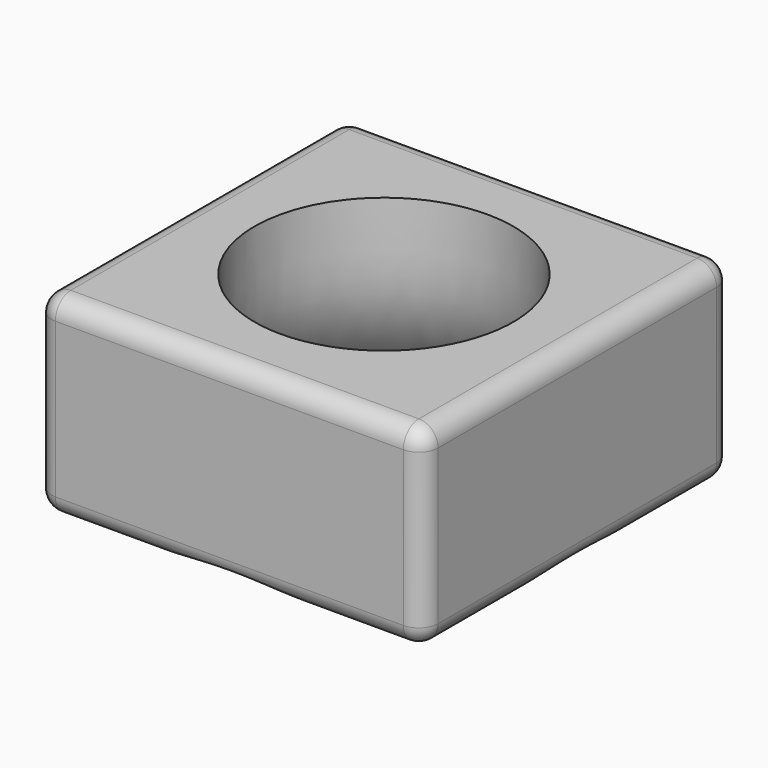
from build123d import *

# Parameters (mm, degrees)
F0_W         = 100
F0_H         = 100
F1_DEPTH     = 50
F4_T1_DEPTH  = 90
F4_T3_DEPTH  = 90
F4_T5_DEPTH  = 74.4845192026
F4_T7_DEPTH  = 74.4484512119
F4_T9_DEPTH  = 74.5795432477
F4_T11_DEPTH = 74.5795432477
F4_T13_DEPTH = 74.3550362655
F4_T15_DEPTH = 74.3550362655
F4_T17_DEPTH = 40
F4_S21_W     = 5
F4_S21_H     = 5
F4_T22_DEPTH = 5
F4_S27_W     = 5
F4_S27_H     = 5
F4_T28_DEPTH = 5
F4_S33_W     = 5
F4_S33_H     = 5
F4_T34_DEPTH = 5
F4_S39_W     = 5
F4_S39_H     = 5
F4_T40_DEPTH = 5
F4_S45_W     = 5
F4_S45_H     = 5
F4_T46_DEPTH = 5
F4_S51_W     = 5
F4_S51_H     = 5
F4_T52_DEPTH = 5
F4_S57_W     = 5
F4_S57_H     = 5
F4_T58_DEPTH = 5
F4_S63_W     = 5
F4_S63_H     = 5
F4_T64_DEPTH = 5


# Not quite as in the source:
# - a fillet or chamfer that OpenCascade refuses, or shapes differently, is made with other operations: its cross-section is extruded or revolved along the edge and cut away or added
# - the dataset's text gives a spline's control points without its knots; the knots are read off the source's solid


with BuildPart() as f1:
    # F0 (on Top) → F1 (new body)
    with BuildSketch(Plane.XY):
        Rectangle(F0_W, F0_H)
    extrude(amount=F1_DEPTH)

    # F2 (on Front) → F3 (revolve, cut)
    with BuildSketch(Plane.XZ):
        with BuildLine():
            Line((-50.0180339954, -0.4668149349), (-0.0180339954, -0.4668149349))
            Line((-0.0180339954, -0.4668149349), (-0.0180339954, 51.5331850651))
            Line((-0.0180339954, 51.5331850651), (-30.0180339954, 51.5331850651))
            Line((-30.0180339954, 51.5331850651), (-33.4886429042, 51.5011279386))
            add(Edge.make_bspline(
                [(-33.4886429042, 51.5011279386), (-33.4950519073, 49.139072917), (-33.3955006037, 44.4370362177), (-33.2935230835, 37.5332689943), (-33.5611952985, 31.9785842308), (-34.168277512, 27.6958965313), (-34.8648891771, 24.5781080346), (-35.8438362297, 21.5436382975), (-37.5227538709, 17.5800116677), (-40.3266208804, 12.746692889), (-44.8284624652, 7.034291652), (-48.5895577258, 3.2216186068), (-50.6592954323, 1.2987297262)],
                knots=[0, 0, 0, 0, 0.125, 0.25, 0.375, 0.4375, 0.5, 0.5625, 0.625, 0.75, 0.875, 1, 1, 1, 1], degree=3))
            Line((-50.6592954323, 1.2987297262), (-50.6592954323, -0.4668149349))
            Line((-50.6592954323, -0.4668149349), (-50.0180339954, -0.4668149349))
        make_face()
    revolve(axis=Axis((-0.0180339954, 0, 25.5331850651), (0, 0, 1)), mode=Mode.SUBTRACT)

    # F4: fillet of radius 5 on 16 edges, made by hand

    # F4_s2 → F4_t1 (cut)
    with BuildSketch(Plane.YZ.offset(-45)):
        with BuildLine():
            ThreePointArc((-45, 50), (-48.5355339059, 48.5355339059), (-50, 45))
            Line((-50, 45), (-50, 50))
            Line((-50, 50), (-45, 50))
        make_face()
        with BuildLine():
            ThreePointArc((50, 45), (48.5355339059, 48.5355339059), (45, 50))
            Line((45, 50), (50, 50))
            Line((50, 50), (50, 45))
        make_face()
    extrude(amount=F4_T1_DEPTH, mode=Mode.SUBTRACT)

    # F4_s4 → F4_t3 (cut)
    with BuildSketch(Plane.XZ.offset(-45)):
        with BuildLine():
            ThreePointArc((-50, 45), (-48.5355339059, 48.5355339059), (-45, 50))
            Line((-45, 50), (-50, 50))
            Line((-50, 50), (-50, 45))
        make_face()
        with BuildLine():
            ThreePointArc((45, 50), (48.5355339059, 48.5355339059), (50, 45))
            Line((50, 45), (50, 50))
            Line((50, 50), (45, 50))
        make_face()
    extrude(amount=F4_T3_DEPTH, mode=Mode.SUBTRACT)

    # F4_s6 → F4_t5 (cut)
    with BuildSketch(Plane.YZ.offset(-29.4845192026)):
        with BuildLine():
            ThreePointArc((-50, 5), (-48.5355339059, 1.4644660941), (-45, 0))
            Line((-45, 0), (-50, 0))
            Line((-50, 0), (-50, 5))
        make_face()
        with BuildLine():
            ThreePointArc((50, 5), (48.5355339059, 1.4644660941), (45, 0))
            Line((45, 0), (50, 0))
            Line((50, 0), (50, 5))
        make_face()
    extrude(amount=F4_T5_DEPTH, mode=Mode.SUBTRACT)

    # F4_s8 → F4_t7 (cut)
    with BuildSketch(Plane.YZ.offset(-45)):
        with BuildLine():
            ThreePointArc((-50, 5), (-48.5355339059, 1.4644660941), (-45, 0))
            Line((-45, 0), (-50, 0))
            Line((-50, 0), (-50, 5))
        make_face()
        with BuildLine():
            ThreePointArc((50, 5), (48.5355339059, 1.4644660941), (45, 0))
            Line((45, 0), (50, 0))
            Line((50, 0), (50, 5))
        make_face()
    extrude(amount=F4_T7_DEPTH, mode=Mode.SUBTRACT)

    # F4_s10 → F4_t9 (cut)
    with BuildSketch(Plane.XZ.offset(-29.5795432477)):
        with BuildLine():
            ThreePointArc((50, 5), (48.5355339059, 1.4644660941), (45, 0))
            Line((45, 0), (50, 0))
            Line((50, 0), (50, 5))
        make_face()
    extrude(amount=F4_T9_DEPTH, mode=Mode.SUBTRACT)

    # F4_s12 → F4_t11 (cut)
    with BuildSketch(Plane.XZ.offset(-45)):
        with BuildLine():
            ThreePointArc((45, 0), (48.5355339059, 1.4644660941), (50, 5))
            Line((50, 5), (50, 0))
            Line((50, 0), (45, 0))
        make_face()
    extrude(amount=F4_T11_DEPTH, mode=Mode.SUBTRACT)

    # F4_s14 → F4_t13 (cut)
    with BuildSketch(Plane.XZ.offset(-45)):
        with BuildLine():
            ThreePointArc((-45, 0), (-48.5355339059, 1.4644660941), (-50, 5))
            Line((-50, 5), (-50, 0))
            Line((-50, 0), (-45, 0))
        make_face()
    extrude(amount=F4_T13_DEPTH, mode=Mode.SUBTRACT)

    # F4_s16 → F4_t15 (cut)
    with BuildSketch(Plane.XZ.offset(-29.3550362655)):
        with BuildLine():
            ThreePointArc((-50, 5), (-48.5355339059, 1.4644660941), (-45, 0))
            Line((-45, 0), (-50, 0))
            Line((-50, 0), (-50, 5))
        make_face()
    extrude(amount=F4_T15_DEPTH, mode=Mode.SUBTRACT)

    # F4_s18 → F4_t17 (cut)
    with BuildSketch(Plane.XY.offset(5)):
        with BuildLine():
            ThreePointArc((50, -45), (48.5355339059, -48.5355339059), (45, -50))
            Line((45, -50), (50, -50))
            Line((50, -50), (50, -45))
        make_face()
        with BuildLine():
            ThreePointArc((-45, 50), (-48.5355339059, 48.5355339059), (-50, 45))
            Line((-50, 45), (-50, 50))
            Line((-50, 50), (-45, 50))
        make_face()
        with BuildLine():
            ThreePointArc((45, 50), (48.5355339059, 48.5355339059), (50, 45))
            Line((50, 45), (50, 50))
            Line((50, 50), (45, 50))
        make_face()
        with BuildLine():
            ThreePointArc((-50, -45), (-48.5355339059, -48.5355339059), (-45, -50))
            Line((-45, -50), (-50, -50))
            Line((-50, -50), (-50, -45))
        make_face()
    extrude(amount=F4_T17_DEPTH, mode=Mode.SUBTRACT)


with BuildPart() as f4_tool20:
    # F4_s21 → F4_t22 (new body)
    with BuildSketch(Plane.XZ.offset(45)):
        with Locations((-47.5, 47.5)):
            Rectangle(F4_S21_W, F4_S21_H)
    extrude(amount=F4_T22_DEPTH)

    # F4_s23 → F4_t24 (revolve, cut)
    with BuildSketch(Plane(origin=(-45, -45, 45), x_dir=(0.7071067812, 0, -0.7071067812), z_dir=(-0.7071067812, 0, -0.7071067812))):
        with BuildLine():
            ThreePointArc((0, -5), (5, 0), (0, 5))
            Line((0, 5), (0, -5))
        make_face()
    revolve(axis=Axis((-45, -45, 45), (0, -1, 0)), mode=Mode.SUBTRACT)


with BuildPart() as f1_1:
    add(f1.part)

    # F4_t19: cut F4_tool20
    add(f4_tool20.part, mode=Mode.SUBTRACT)


with BuildPart() as f4_tool26:
    # F4_s27 → F4_t28 (new body)
    with BuildSketch(Plane.YZ.offset(45)):
        with Locations((-47.5, 47.5)):
            Rectangle(F4_S27_W, F4_S27_H)
    extrude(amount=F4_T28_DEPTH)

    # F4_s29 → F4_t30 (revolve, cut)
    with BuildSketch(Plane(origin=(45, -45, 45), x_dir=(0, 0.7071067812, -0.7071067812), z_dir=(0, -0.7071067812, -0.7071067812))):
        with BuildLine():
            ThreePointArc((0, -5), (5, 0), (0, 5))
            Line((0, 5), (0, -5))
        make_face()
    revolve(axis=Axis((45, -45, 45), (1, 0, 0)), mode=Mode.SUBTRACT)


with BuildPart() as f1_2:
    add(f1_1.part)

    # F4_t25: cut F4_tool26
    add(f4_tool26.part, mode=Mode.SUBTRACT)


with BuildPart() as f4_tool32:
    # F4_s33 → F4_t34 (new body)
    with BuildSketch(Plane.XZ.offset(-45)):
        with Locations((-47.5, 47.5)):
            Rectangle(F4_S33_W, F4_S33_H)
    extrude(amount=-F4_T34_DEPTH)

    # F4_s35 → F4_t36 (revolve, cut)
    with BuildSketch(Plane(origin=(-45, 45, 45), x_dir=(0.7071067812, 0, -0.7071067812), z_dir=(0.7071067812, 0, 0.7071067812))):
        with BuildLine():
            ThreePointArc((0, -5), (5, 0), (0, 5))
            Line((0, 5), (0, -5))
        make_face()
    revolve(axis=Axis((-45, 45, 45), (0, 1, 0)), mode=Mode.SUBTRACT)


with BuildPart() as f1_3:
    add(f1_2.part)

    # F4_t31: cut F4_tool32
    add(f4_tool32.part, mode=Mode.SUBTRACT)


with BuildPart() as f4_tool38:
    # F4_s39 → F4_t40 (new body)
    with BuildSketch(Plane.XZ.offset(-45)):
        with Locations((47.5, 47.5)):
            Rectangle(F4_S39_W, F4_S39_H)
    extrude(amount=-F4_T40_DEPTH)

    # F4_s41 → F4_t42 (revolve, cut)
    with BuildSketch(Plane(origin=(45, 45, 45), x_dir=(-0.7071067812, 0, -0.7071067812), z_dir=(0.7071067812, 0, -0.7071067812))):
        with BuildLine():
            ThreePointArc((0, -5), (5, 0), (0, 5))
            Line((0, 5), (0, -5))
        make_face()
    revolve(axis=Axis((45, 45, 45), (0, 1, 0)), mode=Mode.SUBTRACT)


with BuildPart() as f1_4:
    add(f1_3.part)

    # F4_t37: cut F4_tool38
    add(f4_tool38.part, mode=Mode.SUBTRACT)


with BuildPart() as f4_tool44:
    # F4_s45 → F4_t46 (new body)
    with BuildSketch(Plane.YZ.offset(45)):
        with Locations((-47.5, 2.5)):
            Rectangle(F4_S45_W, F4_S45_H)
    extrude(amount=F4_T46_DEPTH)

    # F4_s47 → F4_t48 (revolve, cut)
    with BuildSketch(Plane(origin=(45, -45, 5), x_dir=(0, 0.7071067812, 0.7071067812), z_dir=(0, 0.7071067812, -0.7071067812))):
        with BuildLine():
            ThreePointArc((0, -5), (5, 0), (0, 5))
            Line((0, 5), (0, -5))
        make_face()
    revolve(axis=Axis((45, -45, 5), (1, 0, 0)), mode=Mode.SUBTRACT)


with BuildPart() as f1_5:
    add(f1_4.part)

    # F4_t43: cut F4_tool44
    add(f4_tool44.part, mode=Mode.SUBTRACT)


with BuildPart() as f4_tool50:
    # F4_s51 → F4_t52 (new body)
    with BuildSketch(Plane.XZ.offset(45)):
        with Locations((-47.5, 2.5)):
            Rectangle(F4_S51_W, F4_S51_H)
    extrude(amount=F4_T52_DEPTH)

    # F4_s53 → F4_t54 (revolve, cut)
    with BuildSketch(Plane(origin=(-45, -45, 5), x_dir=(0.7071067812, 0, 0.7071067812), z_dir=(0.7071067812, 0, -0.7071067812))):
        with BuildLine():
            ThreePointArc((0, -5), (5, 0), (0, 5))
            Line((0, 5), (0, -5))
        make_face()
    revolve(axis=Axis((-45, -45, 5), (0, -1, 0)), mode=Mode.SUBTRACT)


with BuildPart() as f1_6:
    add(f1_5.part)

    # F4_t49: cut F4_tool50
    add(f4_tool50.part, mode=Mode.SUBTRACT)


with BuildPart() as f4_tool56:
    # F4_s57 → F4_t58 (new body)
    with BuildSketch(Plane.YZ.offset(45)):
        with Locations((47.5, 2.5)):
            Rectangle(F4_S57_W, F4_S57_H)
    extrude(amount=F4_T58_DEPTH)

    # F4_s59 → F4_t60 (revolve, cut)
    with BuildSketch(Plane(origin=(45, 45, 5), x_dir=(0, -0.7071067812, 0.7071067812), z_dir=(0, 0.7071067812, 0.7071067812))):
        with BuildLine():
            ThreePointArc((0, -5), (5, 0), (0, 5))
            Line((0, 5), (0, -5))
        make_face()
    revolve(axis=Axis((45, 45, 5), (1, 0, 0)), mode=Mode.SUBTRACT)


with BuildPart() as f1_7:
    add(f1_6.part)

    # F4_t55: cut F4_tool56
    add(f4_tool56.part, mode=Mode.SUBTRACT)


with BuildPart() as f4_tool62:
    # F4_s63 → F4_t64 (new body)
    with BuildSketch(Plane.XZ.offset(-45)):
        with Locations((-47.5, 2.5)):
            Rectangle(F4_S63_W, F4_S63_H)
    extrude(amount=-F4_T64_DEPTH)

    # F4_s65 → F4_t66 (revolve, cut)
    with BuildSketch(Plane(origin=(-45, 45, 5), x_dir=(0.7071067812, 0, 0.7071067812), z_dir=(-0.7071067812, 0, 0.7071067812))):
        with BuildLine():
            ThreePointArc((0, -5), (5, 0), (0, 5))
            Line((0, 5), (0, -5))
        make_face()
    revolve(axis=Axis((-45, 45, 5), (0, 1, 0)), mode=Mode.SUBTRACT)


with BuildPart() as f1_8:
    add(f1_7.part)

    # F4_t61: cut F4_tool62
    add(f4_tool62.part, mode=Mode.SUBTRACT)


solid = f1_8.part
